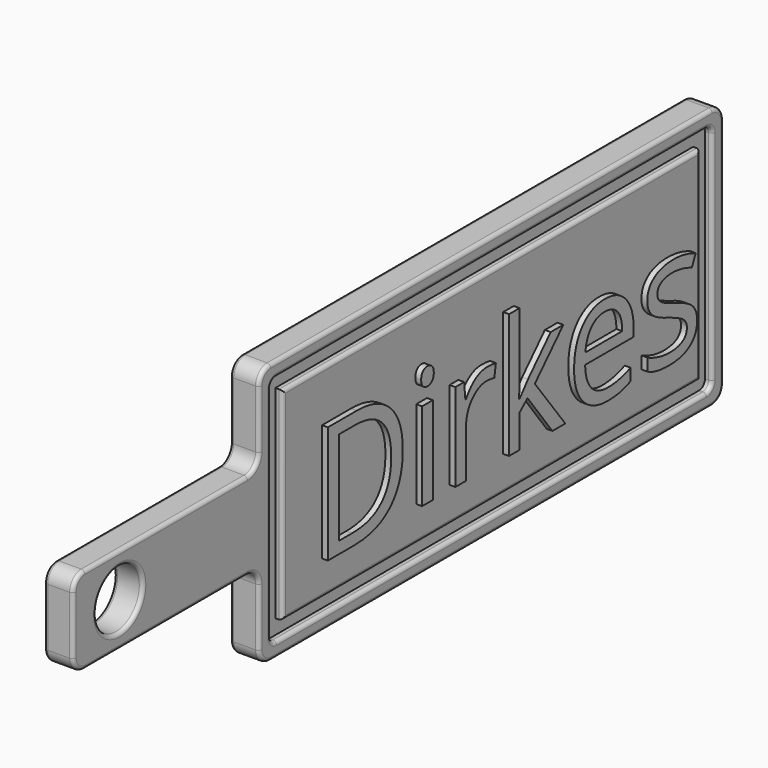
from build123d import *

# Parameters (mm, degrees)
F0_W          = 203.2
F0_H          = 76.2
F1_DEPTH      = 25.4
F2_R          = 25.4
F3_DEPTH      = 25.4
F5_DEPTH      = 6.35
F6_R          = 6.35
F7_R          = 6.35
F8_R          = 6.35
F9_R          = 12.7
F10_R         = 3.175
F11_TEXT_SIZE = 143.7005949103
F12_DEPTH     = 5.08


# Not quite as in the source:
# - Text() gives the source's letters only with a copy of the font that has no kerning and outlines rounded to 1/6400 em; it was checked with that copy


with BuildPart() as f1:
    # F0 (on Right) → F1 (new body)
    with BuildSketch(Plane.YZ):
        Polygon((0, 76.2), (0, 0), (508, 0), (508, 228.6), (0, 228.6), (0, 152.4), align=None)
        with Locations((-101.6, 114.3)):
            Rectangle(F0_W, F0_H)
    extrude(amount=F1_DEPTH)

    # F2 (on face) → F3 (cut)
    with BuildSketch(Plane.YZ.offset(25.4)):
        with Locations((-152.4, 114.3)):
            Circle(F2_R)
    extrude(amount=-F3_DEPTH, mode=Mode.SUBTRACT)

    # F4 (on face) → F5 (cut)
    with BuildSketch(Plane.YZ.offset(25.4)):
        Polygon((12.6999960899, 76.2), (12.6999960899, 12.6999960899), (495.3000039101, 12.6999960899), (495.3000039101, 215.9000039101), (12.6999960899, 215.9000039101), (12.6999960899, 152.4), align=None)
        Polygon((25.6539927483, 76.2), (25.6539927483, 152.4), (25.6539927483, 202.9460072517), (482.3460072517, 202.9460072517), (482.3460072517, 25.6539927483), (25.6539927483, 25.6539927483), align=None, mode=Mode.SUBTRACT)
    extrude(amount=-F5_DEPTH, mode=Mode.SUBTRACT)

    # F6
    f6_edges = [f1.edges().sort_by_distance(p)[0] for p in [
        (22.225, 12.699996, 215.900004),
    ]]
    fillet(f6_edges, radius=F6_R)

    # F7
    f7_edges = [f1.edges().sort_by_distance(p)[0] for p in [
        (22.225, 495.300004, 215.900004),
    ]]
    fillet(f7_edges, radius=F7_R)

    # F8
    f8_edges = [f1.edges().sort_by_distance(p)[0] for p in [
        (22.225, 495.300004, 12.699996),
        (22.225, 12.699996, 12.699996),
    ]]
    fillet(f8_edges, radius=F8_R)

    # F9
    f9_edges = [f1.edges().sort_by_distance(p)[0] for p in [
        (12.7, 0, 228.6),
        (12.7, -203.2, 152.4),
        (12.7, 0, 0),
        (12.7, -203.2, 76.2),
        (12.7, 0, 76.2),
        (12.7, 0, 152.4),
        (12.7, 508, 0),
        (12.7, 508, 228.6),
    ]]
    fillet(f9_edges, radius=F9_R)

    # F10
    f10_edges = [f1.edges().sort_by_distance(p)[0] for p in [
        (25.4, 254, 202.946007),
        (25.4, 482.346007, 114.3),
        (25.4, 254, 25.653993),
        (25.4, 25.653993, 114.3),
        (25.4, 0, 38.1),
        (25.4, -3.719744, 72.480256),
        (25.4, 3.719744, 3.719744),
        (25.4, -101.6, 76.2),
        (25.4, 254, 0),
        (25.4, -199.480256, 79.919744),
        (25.4, 504.280256, 3.719744),
        (25.4, -203.2, 114.3),
        (25.4, 508, 114.3),
        (25.4, -199.480256, 148.680256),
        (25.4, 504.280256, 224.880256),
        (25.4, -101.6, 152.4),
        (25.4, 254, 228.6),
        (25.4, -3.719744, 156.119744),
        (25.4, 3.719744, 224.880256),
        (25.4, 0, 190.5),
        (25.4, 495.300004, 114.3),
        (25.4, 493.440132, 14.559868),
        (25.4, 493.440132, 214.040132),
        (25.4, 254, 12.699996),
        (25.4, 254, 215.900004),
        (25.4, 14.559868, 14.559868),
        (25.4, 14.559868, 214.040132),
        (25.4, 12.699996, 114.3),
        (25.4, -177.8, 114.3),
        (0, 0, 38.1),
        (0, -3.719744, 72.480256),
        (0, 3.719744, 3.719744),
        (0, -101.6, 76.2),
        (0, 254, 0),
        (0, -199.480256, 79.919744),
        (0, 504.280256, 3.719744),
        (0, -203.2, 114.3),
        (0, 508, 114.3),
        (0, -199.480256, 148.680256),
        (0, 504.280256, 224.880256),
        (0, -101.6, 152.4),
        (0, 254, 228.6),
        (0, -3.719744, 156.119744),
        (0, 3.719744, 224.880256),
        (0, 0, 190.5),
        (0, -177.8, 114.3),
    ]]
    fillet(f10_edges, radius=F10_R)

    # F11 (on face) → F12 (join)
    with BuildSketch(Plane.YZ.offset(25.4)):
        with Locations((54.7067187726, 56.2077574432)):
            Text('Dirkes', F11_TEXT_SIZE, font='Open Sans', text_align=(TextAlign.LEFT, TextAlign.BOTTOM))
    extrude(amount=F12_DEPTH)


solid = f1.part
